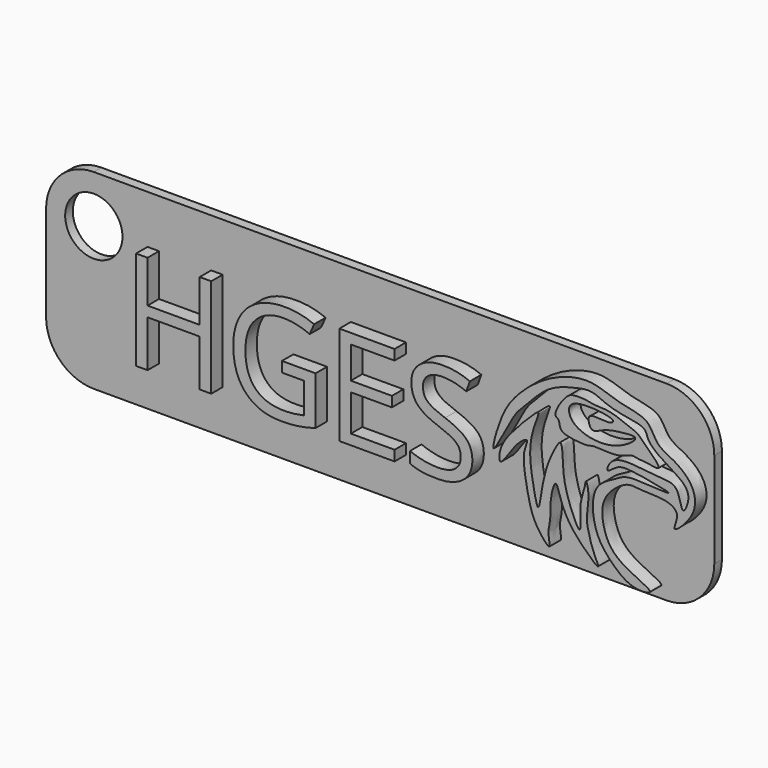
from build123d import *

# Parameters (mm, degrees)
F0_W          = 70
F0_H          = 20
F1_DEPTH      = 1
F4_DEPTH      = 1.5
F6_DEPTH      = 1.5
F8_DEPTH      = 1.5
F10_DEPTH     = 1.5
F11_R         = 5
F12_TEXT_SIZE = 14.5294929906
F13_DEPTH     = 1.5
F2_R          = 3
F14_DEPTH     = 1


# Not quite as in the source:
# - Text() gives the source's letters only with a copy of the font that has no kerning and outlines rounded to 1/6400 em; it was checked with that copy


with BuildPart() as f1:
    # F0 (on Front) → F1 (new body)
    with BuildSketch(Plane.XZ):
        with Locations((10, -1)):
            Rectangle(F0_W, F0_H)
    extrude(amount=-F1_DEPTH)

    # F3 (on face) → F4 (join)
    with BuildSketch(Plane.XZ):
        with BuildLine():
            add(Edge.make_bspline(
                [(23.8162260503, -1.6755688703), (24.1360523759, -0.6575972668), (25.7231504486, 1.0727845273), (28.259531834, 3.7111779221), (27.1372368273, 1.2604371849), (26.7768007825, -1.036938774), (27.1606238788, -3.6081198491), (27.770407849, -6.6093505764), (28.092379912, -4.0735390436), (28.5871570991, -1.7405900159), (29.2988188955, -0.2041079215), (30.280883956, 1.6432138625), (30.3158513257, -1.1386430588), (30.4800656541, -2.4351573269), (30.9185217156, -4.2927695373), (32.4221933191, -7.6159083326), (31.9769895023, -3.9842138731), (32.6213106466, -2.6714026177), (32.7392625928, -1.304503102), (33.185167646, -3.1578190015), (32.6928365856, -4.9828869134), (33.0979990662, -6.6394148726), (33.4656398253, -7.9550270077), (34.4656796969, -9.7961867654), (32.4405554375, -7.9280782136), (31.023194078, -6.3699439418), (30.0941740502, -4.4414986908), (29.5899324739, -2.2918364015), (28.9283722618, -4.7963568366), (29.1226714439, -6.5202052986), (28.6670210741, -7.6919969387), (29.2661867588, -9.7109781903), (27.4816615018, -7.6089620441), (26.8676407752, -5.908760187), (26.3835842843, -3.4466571293), (26.0854993517, -1.1831039262), (26.9188816043, 0.3845016686), (25.2759591602, -0.6322619449), (23.6310977208, -3.7273449289), (23.6366462116, -2.2471515126), (23.8162260503, -1.6755688703)],
                knots=[0, 0, 0, 0, 0.0375977184, 0.0676221393, 0.0913725898, 0.1224880155, 0.1559755773, 0.1829182392, 0.2064966677, 0.2383034913, 0.2652905965, 0.286077174, 0.3126631227, 0.3366740597, 0.3654218498, 0.3941588146, 0.4229386213, 0.4497376699, 0.4659396087, 0.4872886573, 0.5155441792, 0.540289367, 0.5648655583, 0.5859221944, 0.6115391224, 0.6419583046, 0.6716694211, 0.6936890587, 0.7188737585, 0.7459450991, 0.7686011347, 0.7897388087, 0.8152954013, 0.8435507528, 0.8742544016, 0.904647068, 0.924517085, 0.9469653705, 0.9788891918, 1, 1, 1, 1], degree=3))
        make_face()
    extrude(amount=F4_DEPTH)

    # F5 (on face) → F6 (join)
    with BuildSketch(Plane.XZ):
        with BuildLine():
            add(Edge.make_bspline(
                [(23.1035146862, -1.8576275324), (22.9076155792, -1.8805807878), (23.8061852944, 1.5755198099), (25.5415339997, 4.0308552503), (28.6935646366, 6.6776212755), (33.0957147396, 8.0435649543), (36.0951891339, 6.4854228162), (39.4194735036, 6.2527826543), (40.0116112479, 3.9809870698), (42.051772758, 3.2157630609), (44.0848446229, 1.613501515), (44.5298171283, -1.1426105938), (41.3821640982, -4.0242489465), (42.7860863991, -1.4679303199), (40.8813468714, -0.6236041636), (38.4854161464, -0.7697624533), (37.0557943567, -0.3639456276), (34.7981311939, -2.1324024155), (34.385286482, -3.8219492248), (34.576972702, -5.4236481211), (35.5585095298, -8.1436941967), (40.7739741961, -9.8302768518), (37.4537442793, -10.1902093745), (35.3273679598, -8.333773737), (33.5464112146, -6.1999298266), (33.1896449684, -1.7725363423), (35.7815512747, -0.6386186271), (36.9608725155, 0.2175088406), (39.5274599462, 0.0013758493), (42.8364370708, -0.1492163978), (37.246893344, 0.8975794784), (36.0259182222, 0.7404337477), (34.7153550859, -0.4595065059), (35.4586956469, 1.6363301165), (38.6392443758, 1.3059841865), (40.6066773269, 1.0778088252), (42.5459352752, 1.0473069776), (42.7556920441, -1.9884965118), (43.7356084393, 0.1890578413), (43.0487904656, 1.5567304), (40.6881141171, 2.7784950699), (39.1670312587, 4.0913519838), (39.0582829818, 5.206029012), (37.2950814295, 5.5032335229), (34.9910474588, 5.9015041053), (33.40181596, 6.9127519328), (31.3075342871, 6.4281073272), (28.6613933424, 5.7164617469), (26.3467268892, 3.0226703612), (25.2048071027, 2.1672741338), (23.3353482259, -1.8304638842), (23.1035146862, -1.8576275324)],
                knots=[0, 0, 0, 0, 0.0230867257, 0.0484943144, 0.0754557882, 0.1035189007, 0.1282161467, 0.1514731308, 0.1702017075, 0.1895587927, 0.2107131251, 0.2328174803, 0.2546685585, 0.2704151245, 0.2877066454, 0.3088333629, 0.3249150431, 0.3466217865, 0.3640674603, 0.3806336864, 0.403918176, 0.4300455568, 0.4470390931, 0.4700628762, 0.4928231411, 0.5193533365, 0.5403222357, 0.556248946, 0.5789925164, 0.595944393, 0.6227567548, 0.640351186, 0.6535968951, 0.6679875299, 0.691386013, 0.7113521476, 0.7285491871, 0.7467426433, 0.7619278678, 0.7784044401, 0.800454675, 0.8193159489, 0.8319898065, 0.8489101453, 0.8699491481, 0.8879186151, 0.9069385491, 0.9295112929, 0.9537897487, 0.9726783984, 1, 1, 1, 1], degree=3))
        make_face()
    extrude(amount=F6_DEPTH)

    # F7 (on face) → F8 (join)
    with BuildSketch(Plane.XZ):
        with BuildLine():
            add(Edge.make_bspline(
                [(40.3838567436, 1.9684762228), (40.3188861613, 1.7729997946), (39.0358053998, 2.103179936), (38.281093038, 2.0355612872), (37.5102258612, 2.3272022715), (36.203914871, 1.4501126518), (33.4361427557, 1.8522473692), (33.0833649088, 1.5233296454), (30.944317703, 1.6674522746), (29.9611332716, 2.1103662528), (29.9883949717, 3.1057597551), (29.1801788529, 3.1981500805), (30.6096877398, 5.5305343395), (31.5113642081, 5.8139212768), (32.8124769578, 5.7678703919), (33.6018743346, 5.538595812), (35.2220668698, 5.5925325496), (36.905434477, 4.9241020267), (38.2211502181, 4.4387286302), (38.644597536, 3.8633027431), (40.4746029851, 2.2415036538), (40.3838567436, 1.9684762228)],
                knots=[0, 0, 0, 0, 0.0523193321, 0.0972233683, 0.1357096858, 0.1942964674, 0.2705129647, 0.3035325491, 0.3707986249, 0.4186404449, 0.4603818194, 0.4910356637, 0.5620868235, 0.6102422827, 0.6617782411, 0.704941122, 0.7637786461, 0.8286914643, 0.8816043029, 0.9269241159, 1, 1, 1, 1], degree=3))
        make_face()
    extrude(amount=F8_DEPTH)

    # F9 (on face) → F10 (cut)
    with BuildSketch(Plane.XZ.offset(1.5)):
        with BuildLine():
            add(Edge.make_bspline(
                [(35.2548100054, 4.4798986055), (35.499925407, 4.535104446), (36.2148295039, 5.031496094), (31.0781963507, 5.60470284), (30.8506489246, 3.8172753611), (32.0206102152, 2.4999946526), (35.6301800344, 1.9103127944), (38.8221292363, 4.2234795267), (36.2423577821, 3.9463343264), (34.6507705641, 3.7032147831), (33.2719649408, 2.7990632523), (32.8676084396, 4.3181442686), (33.6076502675, 4.6130541536), (34.7789518614, 4.3727239905), (35.2548100054, 4.4798986055)],
                knots=[0, 0, 0, 0, 0.0434781556, 0.1749216123, 0.2461526235, 0.326781116, 0.4531994165, 0.5569030335, 0.6354513569, 0.7268658833, 0.7985484495, 0.8645594129, 0.9155930868, 1, 1, 1, 1], degree=3))
        make_face()
    extrude(amount=-F10_DEPTH, mode=Mode.SUBTRACT)

    # F11
    f11_edges = [f1.edges().sort_by_distance(p)[0] for p in [
        (-25, 0.5, 9),
        (45, 0.5, -11),
        (45, 0.5, 9),
        (-25, 0.5, -11),
    ]]
    fillet(f11_edges, radius=F11_R)

    # F12 (on face) → F13 (join)
    with BuildSketch(Plane.XZ):
        with Locations((-15.8001799136, -6.4499317668)):
            Text('HGES', F12_TEXT_SIZE, font='Open Sans', text_align=(TextAlign.LEFT, TextAlign.BOTTOM))
    extrude(amount=F13_DEPTH)

    # F2 (on face) → F14 (cut, through all)
    with BuildSketch(Plane.XZ):
        with Locations((-20, 4)):
            Circle(F2_R)
    extrude(amount=-F14_DEPTH, mode=Mode.SUBTRACT)


solid = f1.part
